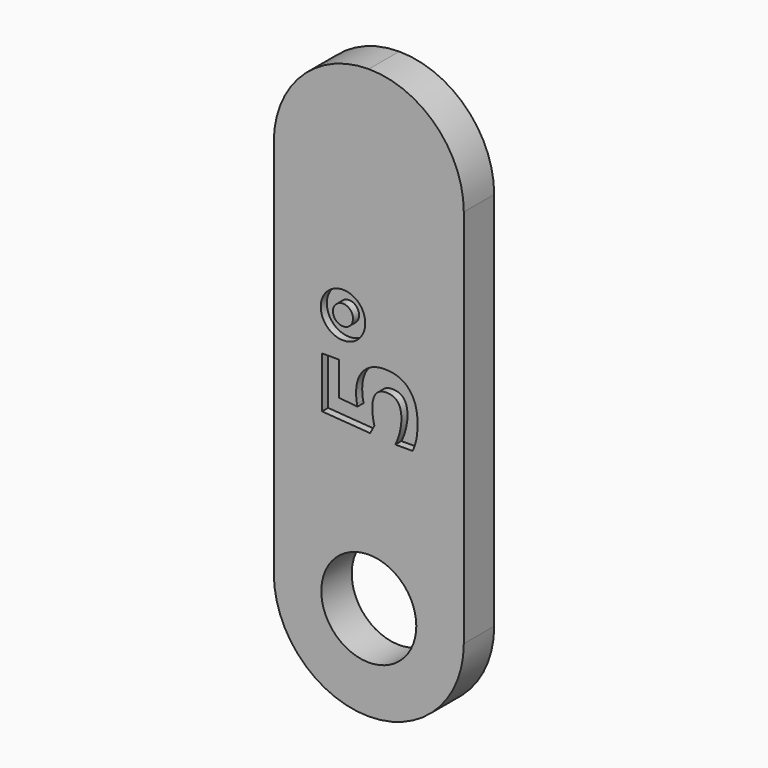
from build123d import *

# Parameters (mm, degrees)
F0_W         = 12.7
F0_H         = 38.1
F0_R         = 3.175
F1_DEPTH     = 2.54
F2_R         = 6.34999
F3_TEXT_SIZE = 8.8194444444
F4_DEPTH     = 0.508


# Not quite as in the source:
# - a fillet or chamfer is up to 0.001 mm smaller than in the source, because OpenCascade refuses the exact size
# - Text() gives the source's letters only with a copy of the font that has no kerning and outlines rounded to 1/6400 em; it was checked with that copy


with BuildPart() as f1:
    # F0 (on Front) → F1 (new body)
    with BuildSketch(Plane.XZ):
        with Locations((6.35, 19.05)):
            Rectangle(F0_W, F0_H)
        with Locations((6.35, 6.35)):
            Circle(F0_R, mode=Mode.SUBTRACT)
    extrude(amount=F1_DEPTH)

    # F2 (radius 6.35 in the source; OpenCascade refuses exactly that, so slightly less here)
    f2_edges = [f1.edges().sort_by_distance(p)[0] for p in [
        (12.7, -1.27, 0),
        (0, -1.27, 0),
        (12.7, -1.27, 38.1),
        (0, -1.27, 38.1),
    ]]
    fillet(f2_edges, radius=F2_R)

    # F3 (on face) → F4 (cut)
    with BuildSketch(Plane.XZ.offset(2.54)):
        with Locations(Location((9.525, 16.1464735243), (0, 0, 90))):
            Text('5°', F3_TEXT_SIZE, font='Open Sans', font_style=FontStyle.BOLD, text_align=(TextAlign.LEFT, TextAlign.BOTTOM))
    extrude(amount=-F4_DEPTH, mode=Mode.SUBTRACT)


solid = f1.part
